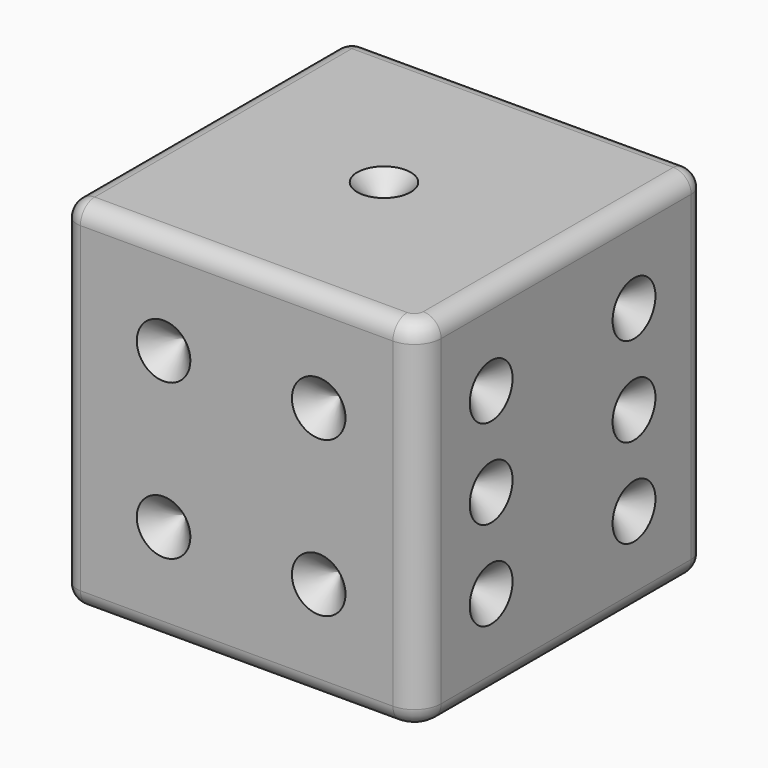
from build123d import *

# Parameters (mm, degrees)
F0_W         = 20
F0_H         = 20
F1_DEPTH     = 20
F2_R         = 1.5
F3_DEPTH     = 1.5
F4_R         = 1.5
F5_DEPTH     = 1.5
F6_R         = 1
F7_SIZE      = 1.49999
F8_R         = 1.5
F9_DEPTH     = 1.5
F10_SIZE     = 1.49999
F11_SIZE     = 1.49999
F12_T1_DEPTH = 20
F12_T4_ANGLE = 90
F12_T6_ANGLE = 90
F13_SIZE     = 1.49999
F14_R        = 1.5
F15_DEPTH    = 1.5
F16_SIZE     = 1.49999
F17_R        = 1.5
F18_DEPTH    = 1.5
F19_SIZE     = 1.49999
F20_R        = 1.5
F21_DEPTH    = 1.5
F22_SIZE     = 1.49999


# Not quite as in the source:
# - a fillet or chamfer that OpenCascade refuses, or shapes differently, is made with other operations: its cross-section is extruded or revolved along the edge and cut away or added
# - a fillet or chamfer is up to 0.001 mm smaller than in the source, because OpenCascade refuses the exact size


with BuildPart() as f1:
    # F0 (on Top) → F1 (new body)
    with BuildSketch(Plane.XY):
        with Locations((10, 10)):
            Rectangle(F0_W, F0_H)
    extrude(amount=F1_DEPTH)

    # F2 (on face) → F3 (cut)
    with BuildSketch(Plane.XY.offset(20)):
        with Locations((10, 10)):
            Circle(F2_R)
    extrude(amount=-F3_DEPTH, mode=Mode.SUBTRACT)

    # F4 (on face) → F5 (cut)
    with BuildSketch(Plane(origin=(0, 20, 0), x_dir=(-1, 0, 0), z_dir=(0, 1, 0))):
        with Locations((-14.3431457505, 14.3431457505)):
            Circle(F4_R)
        with Locations((-5.6568542495, 5.6568542495)):
            Circle(F4_R)
    extrude(amount=-F5_DEPTH, mode=Mode.SUBTRACT)

    # F6
    f6_edges = [f1.edges().sort_by_distance(p)[0] for p in [
        (0, 0, 10),
        (0, 10, 0),
        (20, 20, 10),
        (0, 20, 10),
        (10, 20, 20),
        (0, 10, 20),
        (10, 0, 0),
        (20, 10, 0),
        (20, 10, 20),
        (10, 0, 20),
        (10, 20, 0),
    ]]
    fillet(f6_edges, radius=F6_R)

    # F7 (size 1.5 in the source; OpenCascade refuses exactly that, so slightly less here)
    f7_edges = [f1.edges().sort_by_distance(p)[0] for p in [
        (7.156854, 18.5, 5.656854),
    ]]
    chamfer(f7_edges, length=F7_SIZE)

    # F8 (on face) → F9 (cut)
    with BuildSketch(Plane(origin=(0, 0, 0), x_dir=(1, 0, 0), z_dir=(0, 0, -1))):
        with Locations((5.6568542495, -14.3431457505)):
            Circle(F8_R)
        with Locations((10, -10)):
            Circle(F8_R)
        with Locations((14.3431457505, -5.6568542495)):
            Circle(F8_R)
    extrude(amount=-F9_DEPTH, mode=Mode.SUBTRACT)

    # F10 (size 1.5 in the source; OpenCascade refuses exactly that, so slightly less here)
    f10_edges = [f1.edges().sort_by_distance(p)[0] for p in [
        (15.843146, 18.5, 14.343146),
    ]]
    chamfer(f10_edges, length=F10_SIZE)

    # F11 (size 1.5 in the source; OpenCascade refuses exactly that, so slightly less here)
    f11_edges = [f1.edges().sort_by_distance(p)[0] for p in [
        (8.5, 10, 18.5),
    ]]
    chamfer(f11_edges, length=F11_SIZE)

    # F12: fillet of radius 1.5 on 1 edges, made by hand

    # F12_s2 → F12_t1 (cut)
    with BuildSketch(Plane.XY):
        with BuildLine():
            ThreePointArc((20, 1.5), (19.5606601718, 0.4393398282), (18.5, 0))
            Line((18.5, 0), (20, 0))
            Line((20, 0), (20, 1.5))
        make_face()
    extrude(amount=F12_T1_DEPTH, mode=Mode.SUBTRACT)

    # F12_s3 → F12_t4 (revolve, cut)
    with BuildSketch(Plane.XZ.offset(-1.5)):
        with BuildLine():
            ThreePointArc((19, 0), (19.7071067812, 0.2928932188), (20, 1))
            Line((20, 1), (20, 0))
            Line((20, 0), (19, 0))
        make_face()
    revolve(axis=Axis((18.5, 1.5, 0), (0, 0, -1)), revolution_arc=F12_T4_ANGLE, mode=Mode.SUBTRACT)

    # F12_s5 → F12_t6 (revolve, cut)
    with BuildSketch(Plane.YZ.offset(18.5)):
        with BuildLine():
            ThreePointArc((1, 20), (0.2928932188, 19.7071067812), (0, 19))
            Line((0, 19), (0, 20))
            Line((0, 20), (1, 20))
        make_face()
    revolve(axis=Axis((18.5, 1.5, 20), (0, 0, 1)), revolution_arc=F12_T6_ANGLE, mode=Mode.SUBTRACT)

    # F13 (size 1.5 in the source; OpenCascade refuses exactly that, so slightly less here)
    f13_edges = [f1.edges().sort_by_distance(p)[0] for p in [
        (4.156854, 14.343146, 1.5),
        (8.5, 10, 1.5),
        (12.843146, 5.656854, 1.5),
    ]]
    chamfer(f13_edges, length=F13_SIZE)

    # F14 (on face) → F15 (cut)
    with BuildSketch(Plane.XZ):
        with Locations((5.6568542495, 5.6568542495)):
            Circle(F14_R)
        with Locations((5.6568542495, 14.3431457505)):
            Circle(F14_R)
        with Locations((14.3431457505, 14.3431457505)):
            Circle(F14_R)
        with Locations((14.3431457505, 5.6568542495)):
            Circle(F14_R)
    extrude(amount=-F15_DEPTH, mode=Mode.SUBTRACT)

    # F16 (size 1.5 in the source; OpenCascade refuses exactly that, so slightly less here)
    f16_edges = [f1.edges().sort_by_distance(p)[0] for p in [
        (4.156854, 1.5, 14.343146),
        (12.843146, 1.5, 14.343146),
        (4.156854, 1.5, 5.656854),
        (12.843146, 1.5, 5.656854),
    ]]
    chamfer(f16_edges, length=F16_SIZE)

    # F17 (on face) → F18 (cut)
    with BuildSketch(Plane(origin=(0, 0, 0), x_dir=(0, -1, 0), z_dir=(-1, 0, 0))):
        with Locations((-14.3431457505, 14.3431457505)):
            Circle(F17_R)
        with Locations((-5.7128249468, 14.3996758016)):
            Circle(F17_R)
        with Locations((-10, 10)):
            Circle(F17_R)
        with Locations((-14.3682878079, 5.6818850556)):
            Circle(F17_R)
        with Locations((-5.6568542495, 5.6568542495)):
            Circle(F17_R)
    extrude(amount=-F18_DEPTH, mode=Mode.SUBTRACT)

    # F19 (size 1.5 in the source; OpenCascade refuses exactly that, so slightly less here)
    f19_edges = [f1.edges().sort_by_distance(p)[0] for p in [
        (1.5, 15.843146, 14.343146),
        (1.5, 15.868288, 5.681885),
        (1.5, 11.5, 10),
        (1.5, 7.212825, 14.399676),
        (1.5, 7.156854, 5.656854),
    ]]
    chamfer(f19_edges, length=F19_SIZE)

    # F20 (on face) → F21 (cut)
    with BuildSketch(Plane.YZ.offset(20)):
        with Locations((15, 15)):
            Circle(F20_R)
        with Locations((5, 15)):
            Circle(F20_R)
        with Locations((5, 10)):
            Circle(F20_R)
        with Locations((15, 10)):
            Circle(F20_R)
        with Locations((15, 5)):
            Circle(F20_R)
        with Locations((5, 5)):
            Circle(F20_R)
    extrude(amount=-F21_DEPTH, mode=Mode.SUBTRACT)

    # F22 (size 1.5 in the source; OpenCascade refuses exactly that, so slightly less here)
    f22_edges = [f1.edges().sort_by_distance(p)[0] for p in [
        (18.5, 13.5, 5),
        (18.5, 13.5, 10),
        (18.5, 3.5, 10),
        (18.5, 3.5, 5),
        (18.5, 3.5, 15),
        (18.5, 13.5, 15),
    ]]
    chamfer(f22_edges, length=F22_SIZE)


solid = f1.part
